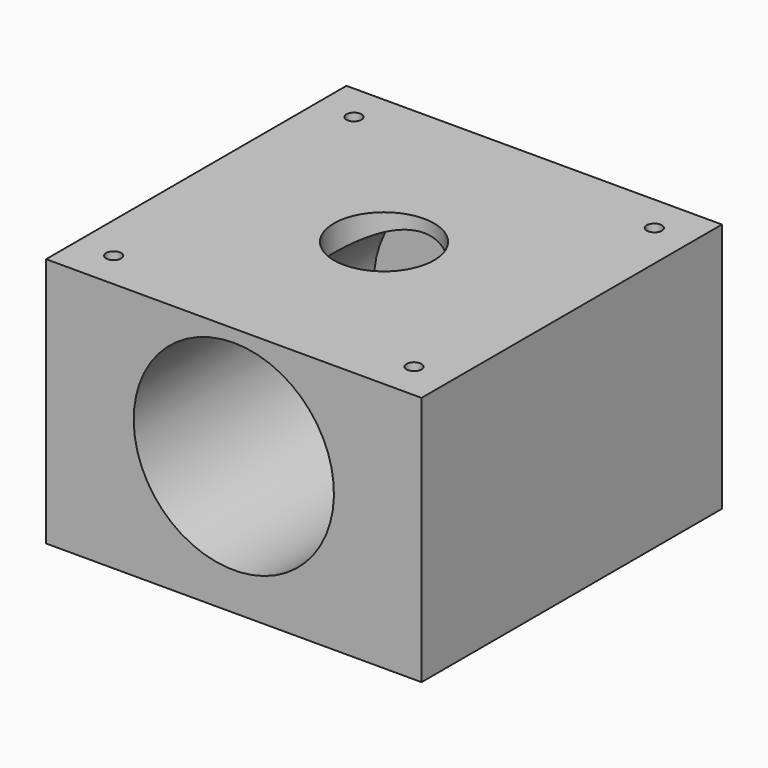
from build123d import *

# Parameters (mm, degrees)
F1_DEPTH  = 2540
F2_W      = 3810
F2_H      = 3810
F2_R      = 508
F3_DEPTH  = 762
F5_DEPTH  = 3048
F7_DEPTH  = 3810.0010001
F8_R      = 254
F9_DEPTH  = 508
F11_DEPTH = 2540.001


with BuildPart() as f1:
    # F0 (on Top) → F1 (new body)
    with BuildSketch(Plane.XY):
        with BuildLine():
            Line((-1905, 0), (0, 0))
            Line((0, 0), (0, 1905))
            Line((0, 1905), (-1397, 1905))
            ThreePointArc((-1397, 1905), (-1545.7897551572, 1545.7897551572), (-1905, 1397))
            Line((-1905, 1397), (-1905, 0))
        make_face()
        with BuildLine():
            Line((-3810, 0), (-1905, 0))
            Line((-1905, 0), (-1905, 1397))
            ThreePointArc((-1905, 1397), (-2264.2102448428, 2264.2102448428), (-1397, 1905))
            Line((-1397, 1905), (0, 1905))
            Line((0, 1905), (0, 3810))
            Line((0, 3810), (-3810, 3810))
            Line((-3810, 3810), (-3810, 0))
        make_face()
    extrude(amount=F1_DEPTH)

    # F2 (on face) → F3 (join)
    with BuildSketch(Plane(origin=(0, 0, 0), x_dir=(1, 0, 0), z_dir=(0, 0, -1))):
        with Locations((-1905, -1905)):
            Rectangle(F2_W, F2_H)
        with Locations((-1905, -1905)):
            Circle(F2_R, mode=Mode.SUBTRACT)
        with Locations((-1905, -1905)):
            Circle(F2_R)
    extrude(amount=-F3_DEPTH)

    # F4 (on face) → F5 (cut)
    with BuildSketch(Plane.XZ):
        with BuildLine():
            ThreePointArc((-889, 1397), (-1186.5795103145, 2115.4204896855), (-1905, 2413))
            ThreePointArc((-1905, 2413), (-2623.4204896855, 678.5795103145), (-889, 1397))
        make_face()
    extrude(amount=-F5_DEPTH, mode=Mode.SUBTRACT)

    # F6 (on face) → F7 (cut, through all)
    with BuildSketch(Plane(origin=(0, 3810, 0), x_dir=(-1, 0, 0), z_dir=(0, 1, 0))):
        with BuildLine():
            ThreePointArc((2159, 1397), (2084.6051224214, 1576.6051224214), (1905, 1651))
            ThreePointArc((1905, 1651), (1725.3948775786, 1217.3948775786), (2159, 1397))
        make_face()
    extrude(amount=-F7_DEPTH, mode=Mode.SUBTRACT)

    # F8 (on face) → F9 (cut)
    with BuildSketch(Plane.XZ.offset(-3048)):
        with Locations((-1905, 1397)):
            Circle(F8_R)
    extrude(amount=-F9_DEPTH, mode=Mode.SUBTRACT)

    # F10 (on face) → F11 (cut, through all)
    with BuildSketch(Plane.XY.offset(2540)):
        with BuildLine():
            ThreePointArc((-3352.8, 3429), (-3375.1184632736, 3482.8815367264), (-3429, 3505.2))
            Line((-3429, 3505.2), (-3429, 3429))
            Line((-3429, 3429), (-3429, 3352.8))
            ThreePointArc((-3429, 3352.8), (-3375.1184632736, 3375.1184632736), (-3352.8, 3429))
        make_face()
        with BuildLine():
            Line((-3429, 3429), (-3429, 3505.2))
            ThreePointArc((-3429, 3505.2), (-3505.2, 3429), (-3429, 3352.8))
            Line((-3429, 3352.8), (-3429, 3429))
        make_face()
        with BuildLine():
            ThreePointArc((-457.2, 3429), (-381, 3352.8), (-304.8, 3429))
            ThreePointArc((-304.8, 3429), (-381, 3505.2), (-457.2, 3429))
        make_face()
        with BuildLine():
            ThreePointArc((-457.2, 381), (-381, 304.8), (-304.8, 381))
            ThreePointArc((-304.8, 381), (-381, 457.2), (-457.2, 381))
        make_face()
        with BuildLine():
            ThreePointArc((-3429, 457.2), (-3482.8815367264, 327.1184632736), (-3352.8, 381))
            ThreePointArc((-3352.8, 381), (-3375.1184632736, 434.8815367264), (-3429, 457.2))
        make_face()
    extrude(amount=-F11_DEPTH, mode=Mode.SUBTRACT)


solid = f1.part
